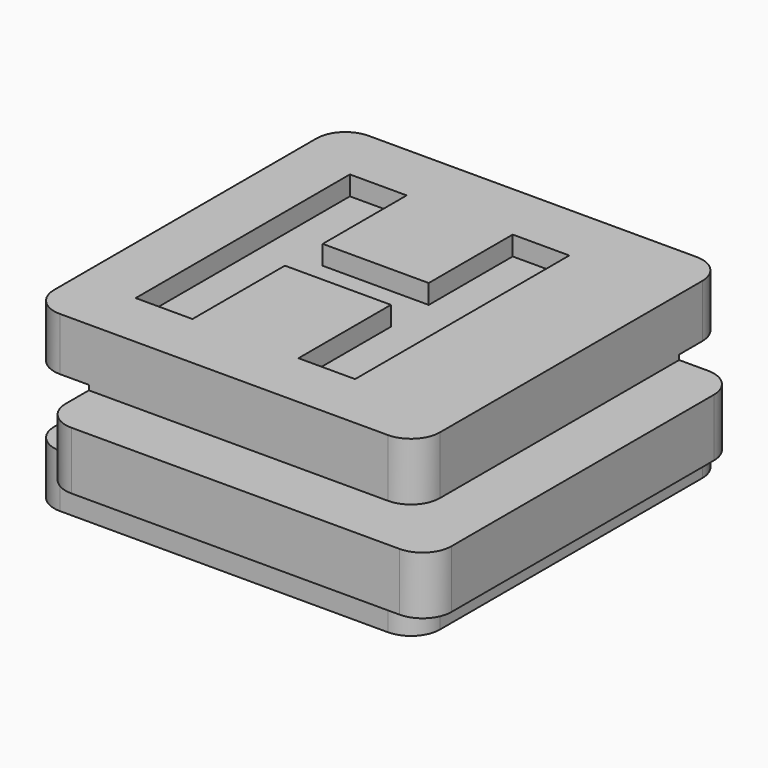
from build123d import *

# Parameters (mm, degrees)
F0_W         = 14
F0_H         = 3
F0_W_2       = 3
F1_DEPTH     = 20
F2_DEPTH     = 3
F3_W         = 3
F3_H         = 3
F4_DEPTH     = 100
F5_W         = 3
F5_H         = 3.5
F6_DEPTH     = 100
F7_R         = 1.5
F8_TEXT_SIZE = 19.4444444444
F9_DEPTH     = 1


# Not quite as in the source:
# - Text() gives the source's letters only with a copy of the font that has no kerning and outlines rounded to 1/6400 em; it was checked with that copy


with BuildPart() as f1:
    # F0 (on Front) → F1 (new body)
    with BuildSketch(Plane.XZ):
        Polygon((10, 1.5), (10, 4.5), (-10, 4.5), (-10, 1.5), (-7, 1.5), (7, 1.5), align=None)
        Rectangle(F0_W, F0_H)
        with Locations((11.5, 0)):
            Rectangle(F0_W_2, F0_H)
        with Locations((8.5, 0)):
            Rectangle(F0_W_2, F0_H)
        with Locations((-8.5, 0)):
            Rectangle(F0_W_2, F0_H)
        Polygon((10, -4.5), (10, -1.5), (7, -1.5), (-7, -1.5), (-10, -1.5), (-10, -4.5), align=None)
    extrude(amount=-F1_DEPTH)

    # F0 (on Front) → F2 (join)
    with BuildSketch(Plane.XZ):
        with Locations((-8.5, 0)):
            Rectangle(F0_W_2, F0_H)
        Rectangle(F0_W, F0_H)
        with Locations((8.5, 0)):
            Rectangle(F0_W_2, F0_H)
        with Locations((11.5, 0)):
            Rectangle(F0_W_2, F0_H)
    extrude(amount=F2_DEPTH)

    # F3 (on face) → F4 (cut)
    with BuildSketch(Plane.YZ.offset(13)):
        Polygon((23, -1.75), (23, 1.75), (17, 1.75), (17, 1.5), (20, 1.5), (20, -1.5), (17, -1.5), (17, -1.75), align=None)
        with Locations((18.5, 0)):
            Rectangle(F3_W, F3_H)
    extrude(amount=-F4_DEPTH, mode=Mode.SUBTRACT)

    # F5 (on face) → F6 (cut)
    with BuildSketch(Plane(origin=(0, 17, 0), x_dir=(-1, 0, 0), z_dir=(0, 1, 0))):
        with Locations((11.5, 0)):
            Rectangle(F5_W, F5_H)
        with Locations((8.5, 0)):
            Rectangle(F5_W, F5_H)
    extrude(amount=-F6_DEPTH, mode=Mode.SUBTRACT)

    # F7
    f7_edges = [f1.edges().sort_by_distance(p)[0] for p in [
        (-7, -3, 0),
        (13, -3, 0),
        (10, 0, 3),
        (10, 0, -3),
        (-10, 0, -3.125),
        (-10, 0, 3.125),
        (-7, 17, 0),
        (-10, 20, 3.125),
        (-10, 20, -3.125),
        (13, 17, 0),
        (10, 20, 3.125),
        (10, 20, -3.125),
    ]]
    fillet(f7_edges, radius=F7_R)

    # F8 (on face) → F9 (cut)
    with BuildSketch(Plane.XY.offset(4.5)):
        with Locations((-8.7207975495, 3)):
            Text('H', F8_TEXT_SIZE, font='Open Sans', font_style=FontStyle.BOLD, text_align=(TextAlign.LEFT, TextAlign.BOTTOM))
    extrude(amount=-F9_DEPTH, mode=Mode.SUBTRACT)


solid = f1.part
